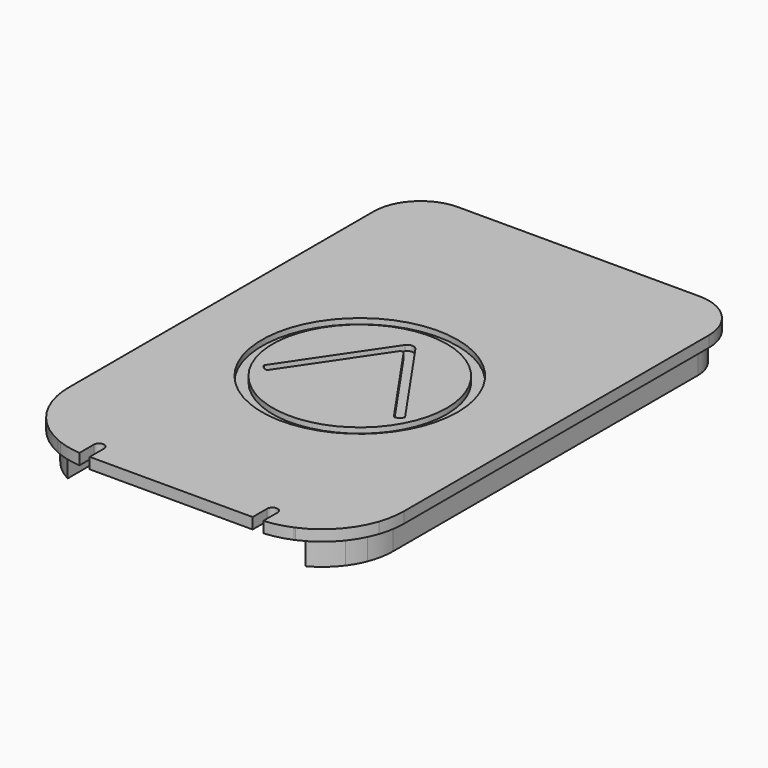
from build123d import *

# Parameters (mm, degrees)
F0_W     = 34.544
F0_H     = 0.2
F0_H_2   = 2
F1_DEPTH = 7.0866
F0_W_2   = 29.673
F2_DEPTH = 2
F0_W_3   = 2.34
F0_H_3   = 4.318
F0_W_4   = 0.2
F3_DEPTH = 7.0866
F4_R     = 17.8300566071
F4_R_2   = 15.8393710275
F5_DEPTH = 1
F6_R     = 1.65
F7_DEPTH = 1.5


with BuildPart() as f1:
    # F0 (on Top) → F1 (new body)
    with BuildSketch(Plane.XY):
        Polygon((12.6492, 41.856), (12.6492, 44.196), (-21.8948, 44.196), (-21.8948, 42.396), (-21.8948, 41.856), align=None)
        with Locations((-4.6228, 44.296)):
            Rectangle(F0_W, F0_H)
        with BuildLine():
            Line((-21.8948, 42.396), (-21.8948, 44.196))
            Line((-21.8948, 44.196), (-21.971, 44.196))
            ThreePointArc((-21.971, 44.196), (-26.4611280605, 42.3361280605), (-28.321, 37.846))
            Line((-28.321, 37.846), (-28.321, -31.496))
            ThreePointArc((-28.321, -31.496), (-28.0890375223, -33.9122037045), (-27.4016235683, -36.2401446376))
            Line((-27.4016235683, -36.2401446376), (-25.981, -36.2401446376))
            Line((-25.981, -36.2401446376), (-25.981, -31.496))
            Line((-25.981, -31.496), (-25.981, 37.846))
            ThreePointArc((-25.981, 37.846), (-24.8064981926, 40.6814981926), (-21.971, 41.856))
            Line((-21.971, 41.856), (-21.8948, 41.856))
            Line((-21.8948, 41.856), (-21.8948, 42.396))
        make_face()
        with Locations((-4.6228, 45.396)):
            Rectangle(F0_W, F0_H_2)
    extrude(amount=-F1_DEPTH)

    # F0 (on Top) → F2 (join)
    with BuildSketch(Plane.XY):
        with BuildLine():
            Line((12.6492, 46.396), (12.6492, 44.396))
            Line((12.6492, 44.396), (21.971, 44.396))
            ThreePointArc((21.971, 44.396), (26.6025494168, 42.4775494168), (28.521, 37.846))
            Line((28.521, 37.846), (28.521, 33.8582))
            Line((28.521, 33.8582), (28.521, 29.5402))
            Line((28.521, 29.5402), (28.521, -31.496))
            ThreePointArc((28.521, -31.496), (28.2929750434, -33.910756406), (27.6169614728, -36.2401446376))
            Line((27.6169614728, -36.2401446376), (29.7455563349, -36.2401446376))
            ThreePointArc((29.7455563349, -36.2401446376), (30.3258612606, -33.8995505622), (30.521, -31.496))
            Line((30.521, -31.496), (30.521, 37.846))
            ThreePointArc((30.521, 37.846), (28.0167629791, 43.8917629791), (21.971, 46.396))
            Line((21.971, 46.396), (12.6492, 46.396))
        make_face()
        with BuildLine():
            ThreePointArc((16.7415, -46.3538087129), (19.1412490439, -45.9741851994), (21.4474, -45.2096086804))
            Line((21.4474, -45.2096086804), (21.4474, -43.0052598824))
            ThreePointArc((21.4474, -43.0052598824), (19.1586666659, -43.9014389105), (16.7415, -44.347244288))
            Line((16.7415, -44.347244288), (16.7415, -46.3538087129))
        make_face()
        with BuildLine():
            Line((21.971, 41.856), (12.6492, 41.856))
            Line((12.6492, 41.856), (-21.8948, 41.856))
            Line((-21.8948, 41.856), (-21.971, 41.856))
            ThreePointArc((-21.971, 41.856), (-24.8064981926, 40.6814981926), (-25.981, 37.846))
            Line((-25.981, 37.846), (-25.981, -31.496))
            ThreePointArc((-25.981, -31.496), (-25.6893764307, -33.9367777552), (-24.8309235424, -36.2401446376))
            Line((-24.8309235424, -36.2401446376), (-21.631, -36.2401446376))
            Line((-21.631, -36.2401446376), (-21.631, -39.9345721541))
            ThreePointArc((-21.631, -39.9345721541), (-18.7758369596, -41.3639584392), (-15.621, -41.856))
            Line((-15.621, -41.856), (15.621, -41.856))
            ThreePointArc((15.621, -41.856), (18.7758369596, -41.3639584392), (21.631, -39.9345721541))
            Line((21.631, -39.9345721541), (21.631, -36.2401446376))
            Line((21.631, -36.2401446376), (24.8309235424, -36.2401446376))
            ThreePointArc((24.8309235424, -36.2401446376), (25.6893764307, -33.9367777552), (25.981, -31.496))
            Line((25.981, -31.496), (25.981, 29.5402))
            Line((25.981, 29.5402), (25.981, 33.8582))
            Line((25.981, 33.8582), (25.981, 37.846))
            ThreePointArc((25.981, 37.846), (24.8064981926, 40.6814981926), (21.971, 41.856))
        make_face()
        with Locations((0, -45.396)):
            Rectangle(F0_W_2, F0_H_2)
        with BuildLine():
            Line((-21.971, 44.396), (-21.8948, 44.396))
            Line((-21.8948, 44.396), (-21.8948, 46.396))
            Line((-21.8948, 46.396), (-21.971, 46.396))
            ThreePointArc((-21.971, 46.396), (-28.0167629791, 43.8917629791), (-30.521, 37.846))
            Line((-30.521, 37.846), (-30.521, -31.496))
            ThreePointArc((-30.521, -31.496), (-30.3258612606, -33.8995505622), (-29.7455563349, -36.2401446376))
            Line((-29.7455563349, -36.2401446376), (-27.6169614728, -36.2401446376))
            ThreePointArc((-27.6169614728, -36.2401446376), (-28.2929750434, -33.910756406), (-28.521, -31.496))
            Line((-28.521, -31.496), (-28.521, 37.846))
            ThreePointArc((-28.521, 37.846), (-26.6025494168, 42.4775494168), (-21.971, 44.396))
        make_face()
        with Locations((0, -44.296)):
            Rectangle(F0_W_2, F0_H)
        with BuildLine():
            Line((-16.7415, -46.3538087129), (-16.7415, -44.347244288))
            ThreePointArc((-16.7415, -44.347244288), (-18.9035466854, -43.9713712273), (-20.9706, -43.2344743404))
            Line((-20.9706, -43.2344743404), (-20.9706, -45.4025373059))
            ThreePointArc((-20.9706, -45.4025373059), (-18.8908284091, -46.0327885785), (-16.7415, -46.3538087129))
        make_face()
        with BuildLine():
            Line((21.631, -42.9104601274), (21.631, -42.6839354664))
            ThreePointArc((21.631, -42.6839354664), (19.2604727553, -43.663343098), (16.7415, -44.146473499))
            Line((16.7415, -44.146473499), (16.7415, -44.347244288))
            ThreePointArc((16.7415, -44.347244288), (19.1586666659, -43.9014389105), (21.4474, -43.0052598824))
            ThreePointArc((21.4474, -43.0052598824), (21.5393898138, -42.95822762), (21.631, -42.9104601274))
        make_face()
        with BuildLine():
            ThreePointArc((16.7415, -44.146473499), (19.2604727553, -43.663343098), (21.631, -42.6839354664))
            Line((21.631, -42.6839354664), (21.631, -39.9345721541))
            ThreePointArc((21.631, -39.9345721541), (18.7758369596, -41.3639584392), (15.621, -41.856))
            Line((15.621, -41.856), (-15.621, -41.856))
            ThreePointArc((-15.621, -41.856), (-18.7758369596, -41.3639584392), (-21.631, -39.9345721541))
            Line((-21.631, -39.9345721541), (-21.631, -42.6839354664))
            ThreePointArc((-21.631, -42.6839354664), (-19.2604727553, -43.663343098), (-16.7415, -44.146473499))
            Line((-16.7415, -44.146473499), (-16.7415, -43.094))
            ThreePointArc((-16.7415, -43.094), (-15.789, -42.1415), (-14.8365, -43.094))
            Line((-14.8365, -43.094), (-14.8365, -44.196))
            Line((-14.8365, -44.196), (14.8365, -44.196))
            Line((14.8365, -44.196), (14.8365, -43.094))
            ThreePointArc((14.8365, -43.094), (15.789, -42.1415), (16.7415, -43.094))
            Line((16.7415, -43.094), (16.7415, -44.146473499))
        make_face()
        with BuildLine():
            Line((29.7455563349, -36.2401446376), (27.6169614728, -36.2401446376))
            ThreePointArc((27.6169614728, -36.2401446376), (26.8953708022, -37.7648565954), (25.981, -39.1823775603))
            ThreePointArc((25.981, -39.1823775603), (24.0155741349, -41.2909540628), (21.631, -42.9104601274))
            Line((21.631, -42.9104601274), (21.631, -45.1301446376))
            ThreePointArc((21.631, -45.1301446376), (26.6259132073, -41.5409930463), (29.7455563349, -36.2401446376))
        make_face()
        with BuildLine():
            ThreePointArc((21.631, -39.9345721541), (23.4519461004, -38.2787636825), (24.8309235424, -36.2401446376))
            Line((24.8309235424, -36.2401446376), (21.631, -36.2401446376))
            Line((21.631, -36.2401446376), (21.631, -39.9345721541))
        make_face()
        with BuildLine():
            Line((-21.631, -36.2401446376), (-24.8309235424, -36.2401446376))
            ThreePointArc((-24.8309235424, -36.2401446376), (-23.4519461004, -38.2787636825), (-21.631, -39.9345721541))
            Line((-21.631, -39.9345721541), (-21.631, -36.2401446376))
        make_face()
        with BuildLine():
            ThreePointArc((-25.981, -39.1823775603), (-26.8953708022, -37.7648565954), (-27.6169614728, -36.2401446376))
            Line((-27.6169614728, -36.2401446376), (-29.7455563349, -36.2401446376))
            ThreePointArc((-29.7455563349, -36.2401446376), (-26.6259132073, -41.5409930463), (-21.631, -45.1301446376))
            Line((-21.631, -45.1301446376), (-21.631, -42.9104601274))
            ThreePointArc((-21.631, -42.9104601274), (-24.0155741349, -41.2909540628), (-25.981, -39.1823775603))
        make_face()
        with BuildLine():
            ThreePointArc((-20.9706, -43.2344743404), (-21.3031100256, -43.0771754869), (-21.631, -42.9104601274))
            Line((-21.631, -42.9104601274), (-21.631, -45.1301446376))
            ThreePointArc((-21.631, -45.1301446376), (-21.3024326962, -45.2702993476), (-20.9706, -45.4025373059))
            Line((-20.9706, -45.4025373059), (-20.9706, -43.2344743404))
        make_face()
        with BuildLine():
            ThreePointArc((21.4474, -45.2096086804), (21.5393333696, -45.1701848067), (21.631, -45.1301446376))
            Line((21.631, -45.1301446376), (21.631, -42.9104601274))
            ThreePointArc((21.631, -42.9104601274), (21.5393898138, -42.95822762), (21.4474, -43.0052598824))
            Line((21.4474, -43.0052598824), (21.4474, -45.2096086804))
        make_face()
        with BuildLine():
            ThreePointArc((-16.7415, -44.146473499), (-19.2604727553, -43.663343098), (-21.631, -42.6839354664))
            Line((-21.631, -42.6839354664), (-21.631, -42.9104601274))
            ThreePointArc((-21.631, -42.9104601274), (-21.3031100256, -43.0771754869), (-20.9706, -43.2344743404))
            ThreePointArc((-20.9706, -43.2344743404), (-18.9035466854, -43.9713712273), (-16.7415, -44.347244288))
            Line((-16.7415, -44.347244288), (-16.7415, -44.146473499))
        make_face()
    extrude(amount=-F2_DEPTH)

    # F0 (on Top) → F3 (join)
    with BuildSketch(Plane.XY):
        with BuildLine():
            Line((-21.8948, 42.396), (-21.8948, 44.196))
            Line((-21.8948, 44.196), (-21.971, 44.196))
            ThreePointArc((-21.971, 44.196), (-26.4611280605, 42.3361280605), (-28.321, 37.846))
            Line((-28.321, 37.846), (-28.321, -31.496))
            ThreePointArc((-28.321, -31.496), (-28.0890375223, -33.9122037045), (-27.4016235683, -36.2401446376))
            Line((-27.4016235683, -36.2401446376), (-25.981, -36.2401446376))
            Line((-25.981, -36.2401446376), (-25.981, -31.496))
            Line((-25.981, -31.496), (-25.981, 37.846))
            ThreePointArc((-25.981, 37.846), (-24.8064981926, 40.6814981926), (-21.971, 41.856))
            Line((-21.971, 41.856), (-21.8948, 41.856))
            Line((-21.8948, 41.856), (-21.8948, 42.396))
        make_face()
        with BuildLine():
            ThreePointArc((28.321, 37.846), (26.4611280605, 42.3361280605), (21.971, 44.196))
            Line((21.971, 44.196), (12.6492, 44.196))
            Line((12.6492, 44.196), (12.6492, 41.856))
            Line((12.6492, 41.856), (21.971, 41.856))
            ThreePointArc((21.971, 41.856), (24.8064981926, 40.6814981926), (25.981, 37.846))
            Line((25.981, 37.846), (25.981, 33.8582))
            Line((25.981, 33.8582), (28.321, 33.8582))
            Line((28.321, 33.8582), (28.321, 37.846))
        make_face()
        with Locations((27.151, 31.6992)):
            Rectangle(F0_W_3, F0_H_3)
        with BuildLine():
            Line((28.321, -31.496), (28.321, 29.5402))
            Line((28.321, 29.5402), (25.981, 29.5402))
            Line((25.981, 29.5402), (25.981, -31.496))
            Line((25.981, -31.496), (25.981, -36.2401446376))
            Line((25.981, -36.2401446376), (27.4016235683, -36.2401446376))
            ThreePointArc((27.4016235683, -36.2401446376), (28.0890375223, -33.9122037045), (28.321, -31.496))
        make_face()
        with BuildLine():
            Line((12.6492, 44.196), (21.971, 44.196))
            ThreePointArc((21.971, 44.196), (26.4611280605, 42.3361280605), (28.321, 37.846))
            Line((28.321, 37.846), (28.321, 33.8582))
            Line((28.321, 33.8582), (28.521, 33.8582))
            Line((28.521, 33.8582), (28.521, 37.846))
            ThreePointArc((28.521, 37.846), (26.6025494168, 42.4775494168), (21.971, 44.396))
            Line((21.971, 44.396), (12.6492, 44.396))
            Line((12.6492, 44.396), (12.6492, 44.196))
        make_face()
        with Locations((28.421, 31.6992)):
            Rectangle(F0_W_4, F0_H_3)
        with BuildLine():
            Line((28.521, 29.5402), (28.321, 29.5402))
            Line((28.321, 29.5402), (28.321, -31.496))
            ThreePointArc((28.321, -31.496), (28.0890375223, -33.9122037045), (27.4016235683, -36.2401446376))
            Line((27.4016235683, -36.2401446376), (27.6169614728, -36.2401446376))
            ThreePointArc((27.6169614728, -36.2401446376), (28.2929750434, -33.910756406), (28.521, -31.496))
            Line((28.521, -31.496), (28.521, 29.5402))
        make_face()
        with BuildLine():
            Line((-21.971, 44.196), (-21.8948, 44.196))
            Line((-21.8948, 44.196), (-21.8948, 44.396))
            Line((-21.8948, 44.396), (-21.971, 44.396))
            ThreePointArc((-21.971, 44.396), (-26.6025494168, 42.4775494168), (-28.521, 37.846))
            Line((-28.521, 37.846), (-28.521, -31.496))
            ThreePointArc((-28.521, -31.496), (-28.2929750434, -33.910756406), (-27.6169614728, -36.2401446376))
            Line((-27.6169614728, -36.2401446376), (-27.4016235683, -36.2401446376))
            ThreePointArc((-27.4016235683, -36.2401446376), (-28.0890375223, -33.9122037045), (-28.321, -31.496))
            Line((-28.321, -31.496), (-28.321, 37.846))
            ThreePointArc((-28.321, 37.846), (-26.4611280605, 42.3361280605), (-21.971, 44.196))
        make_face()
        with BuildLine():
            ThreePointArc((-24.8309235424, -36.2401446376), (-25.6893764307, -33.9367777552), (-25.981, -31.496))
            Line((-25.981, -31.496), (-25.981, -36.2401446376))
            Line((-25.981, -36.2401446376), (-24.8309235424, -36.2401446376))
        make_face()
        with BuildLine():
            Line((-25.981, -36.2401446376), (-27.4016235683, -36.2401446376))
            ThreePointArc((-27.4016235683, -36.2401446376), (-26.7674757756, -37.5825489223), (-25.981, -38.8417742955))
            Line((-25.981, -38.8417742955), (-25.981, -36.2401446376))
        make_face()
        with BuildLine():
            Line((-25.981, -36.2401446376), (-25.981, -38.8417742955))
            ThreePointArc((-25.981, -38.8417742955), (-24.0284238394, -41.0146776594), (-21.631, -42.6839354664))
            Line((-21.631, -42.6839354664), (-21.631, -39.9345721541))
            ThreePointArc((-21.631, -39.9345721541), (-23.4519461004, -38.2787636825), (-24.8309235424, -36.2401446376))
            Line((-24.8309235424, -36.2401446376), (-25.981, -36.2401446376))
        make_face()
        with BuildLine():
            Line((-21.631, -36.2401446376), (-24.8309235424, -36.2401446376))
            ThreePointArc((-24.8309235424, -36.2401446376), (-23.4519461004, -38.2787636825), (-21.631, -39.9345721541))
            Line((-21.631, -39.9345721541), (-21.631, -36.2401446376))
        make_face()
        with BuildLine():
            ThreePointArc((-25.981, -38.8417742955), (-26.7674757756, -37.5825489223), (-27.4016235683, -36.2401446376))
            Line((-27.4016235683, -36.2401446376), (-27.6169614728, -36.2401446376))
            ThreePointArc((-27.6169614728, -36.2401446376), (-26.8953708022, -37.7648565954), (-25.981, -39.1823775603))
            Line((-25.981, -39.1823775603), (-25.981, -38.8417742955))
        make_face()
        with BuildLine():
            ThreePointArc((-21.631, -42.6839354664), (-24.0284238394, -41.0146776594), (-25.981, -38.8417742955))
            Line((-25.981, -38.8417742955), (-25.981, -39.1823775603))
            ThreePointArc((-25.981, -39.1823775603), (-24.0155741349, -41.2909540628), (-21.631, -42.9104601274))
            Line((-21.631, -42.9104601274), (-21.631, -42.6839354664))
        make_face()
        with BuildLine():
            Line((25.981, -36.2401446376), (25.981, -31.496))
            ThreePointArc((25.981, -31.496), (25.6893764307, -33.9367777552), (24.8309235424, -36.2401446376))
            Line((24.8309235424, -36.2401446376), (25.981, -36.2401446376))
        make_face()
        with BuildLine():
            ThreePointArc((25.981, -38.8417742955), (26.7674757756, -37.5825489223), (27.4016235683, -36.2401446376))
            Line((27.4016235683, -36.2401446376), (25.981, -36.2401446376))
            Line((25.981, -36.2401446376), (25.981, -38.8417742955))
        make_face()
        with BuildLine():
            ThreePointArc((21.631, -42.6839354664), (24.0284238394, -41.0146776594), (25.981, -38.8417742955))
            Line((25.981, -38.8417742955), (25.981, -36.2401446376))
            Line((25.981, -36.2401446376), (24.8309235424, -36.2401446376))
            ThreePointArc((24.8309235424, -36.2401446376), (23.4519461004, -38.2787636825), (21.631, -39.9345721541))
            Line((21.631, -39.9345721541), (21.631, -42.6839354664))
        make_face()
        with BuildLine():
            Line((25.981, -39.1823775603), (25.981, -38.8417742955))
            ThreePointArc((25.981, -38.8417742955), (24.0284238394, -41.0146776594), (21.631, -42.6839354664))
            Line((21.631, -42.6839354664), (21.631, -42.9104601274))
            ThreePointArc((21.631, -42.9104601274), (24.0155741349, -41.2909540628), (25.981, -39.1823775603))
        make_face()
        with BuildLine():
            Line((27.6169614728, -36.2401446376), (27.4016235683, -36.2401446376))
            ThreePointArc((27.4016235683, -36.2401446376), (26.7674757756, -37.5825489223), (25.981, -38.8417742955))
            Line((25.981, -38.8417742955), (25.981, -39.1823775603))
            ThreePointArc((25.981, -39.1823775603), (26.8953708022, -37.7648565954), (27.6169614728, -36.2401446376))
        make_face()
        with BuildLine():
            ThreePointArc((21.631, -39.9345721541), (23.4519461004, -38.2787636825), (24.8309235424, -36.2401446376))
            Line((24.8309235424, -36.2401446376), (21.631, -36.2401446376))
            Line((21.631, -36.2401446376), (21.631, -39.9345721541))
        make_face()
    extrude(amount=-F3_DEPTH)

    # F4 (on face) → F5 (cut)
    with BuildSketch(Plane.XY):
        with Locations((-0.4097813458, -2.9451847493)):
            Circle(F4_R)
        with Locations((-0.4097813458, -2.9451847493)):
            Circle(F4_R_2, mode=Mode.SUBTRACT)
        with BuildLine():
            ThreePointArc((0.5613541242, 8.5083885599), (-0.4056551824, 9.0128094008), (-1.3680046302, 8.4995541776))
            Line((-1.3680046302, 8.4995541776), (-13.1364011854, -8.8710766702))
            ThreePointArc((-13.1364011854, -8.8710766702), (-12.6284368081, -9.5223845688), (-11.8442001663, -9.7816193603))
            Line((-11.8442001663, -9.7816193603), (-0.8209832597, 6.4890960886))
            ThreePointArc((-0.8209832597, 6.4890960886), (-0.4080106872, 6.7093490647), (0.0069615684, 6.492887183))
            Line((0.0069615684, 6.492887183), (11.2515560359, -9.7816193603))
            ThreePointArc((11.2515560359, -9.7816193603), (12.050834777, -9.5294881376), (12.5694010689, -8.8710766702))
            Line((12.5694010689, -8.8710766702), (0.5613541242, 8.5083885599))
        make_face()
    extrude(amount=-F5_DEPTH, mode=Mode.SUBTRACT)

    # F6 (on face) → F7 (cut)
    with BuildSketch(Plane(origin=(0, 0, -2), x_dir=(1, 0, 0), z_dir=(0, 0, -1))):
        with Locations((-17.0656, -21.7392)):
            Circle(F6_R)
        with Locations((-13.5096, -21.7392)):
            Circle(F6_R)
        with Locations((16.7164, -21.7392)):
            Circle(F6_R)
    extrude(amount=-F7_DEPTH, mode=Mode.SUBTRACT)


solid = f1.part
